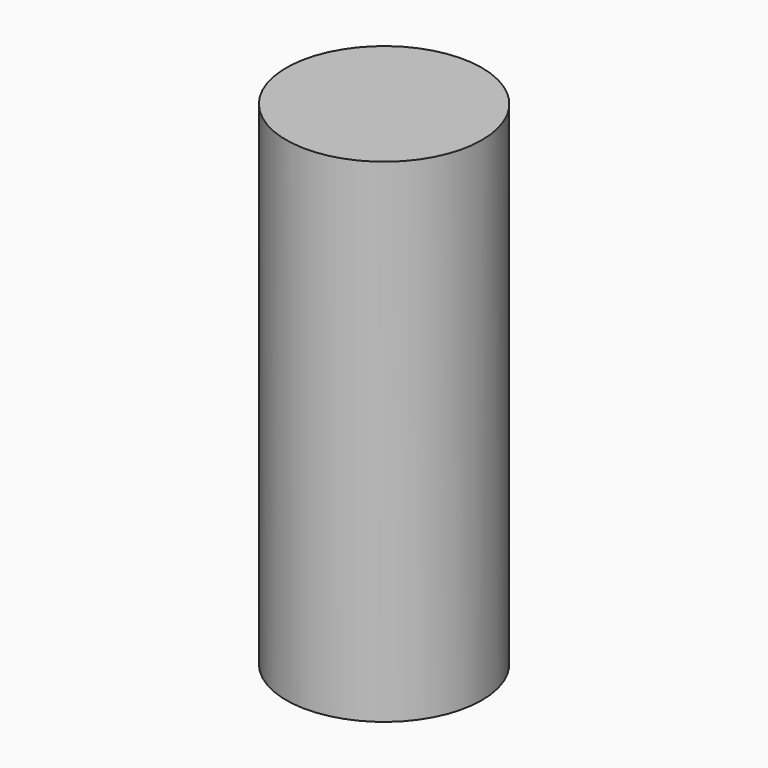
from build123d import *

# Parameters (mm, degrees)
F0_R     = 10.0787403768
F2_DEPTH = 50.8


# Not quite as in the source:
# - a variable given as a bare number and used for a length is read in inches; the dataset says mm whatever the document's units were


with BuildPart() as f2:
    # F0 (on Top) → F2 (new body)
    with BuildSketch(Plane.XY):
        Circle(F0_R)
    extrude(amount=F2_DEPTH)


solid = f2.part
